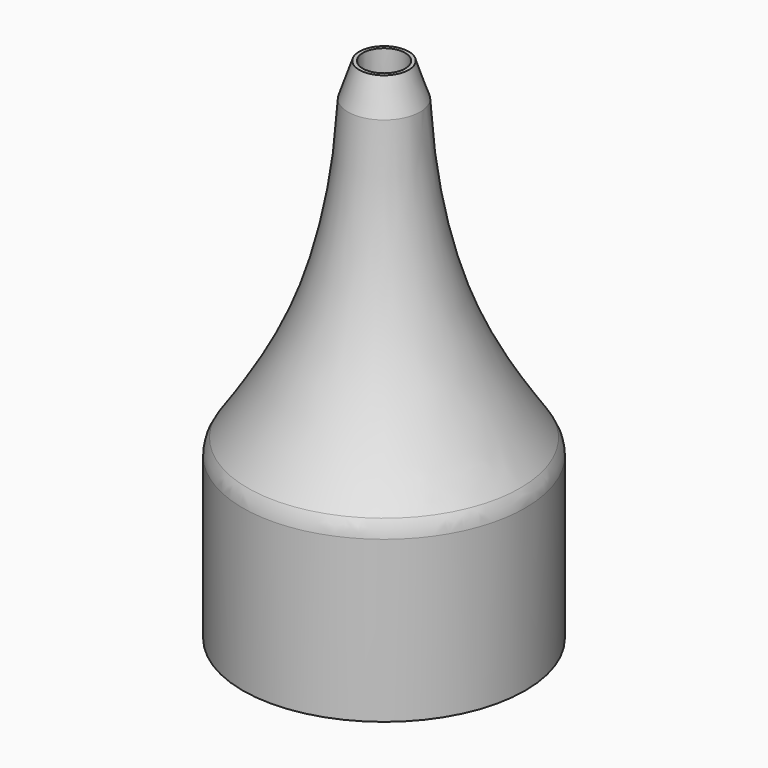
from build123d import *

# Parameters (mm, degrees)
F2_R = 6.35
F3_R = 3.175


# Not quite as in the source:
# - a fillet or chamfer that OpenCascade refuses, or shapes differently, is made with other operations: its cross-section is extruded or revolved along the edge and cut away or added


with BuildPart() as f1:
    # F0 (on Front) → F1 (revolve)
    with BuildSketch(Plane.XZ):
        with BuildLine():
            Line((28.575, 37.618366381), (28.575, 0))
            Line((28.575, 0), (31.75, 0))
            Line((31.75, 0), (31.75, 38.1))
            add(Edge.make_bspline(
                [(31.75, 38.1), (25.5696352748, 47.053791559), (12.6494179223, 66.7292187435), (7.9375, 97.4673148441), (7.9375, 114.3)],
                knots=[0, 0, 0, 0, 0.4558311814, 1, 1, 1, 1], degree=3))
            Line((7.9375, 114.3), (4.7625, 114.3))
            add(Edge.make_bspline(
                [(28.575, 37.618366381), (22.2120435784, 45.9360541366), (8.4198305726, 64.5807348307), (4.7625, 96.5429267445), (4.7625, 114.3)],
                knots=[0, 0, 0, 0, 0.4464692499, 1, 1, 1, 1], degree=3))
        make_face()
    revolve(axis=Axis((0, 0, 57.15), (0, 0, 1)))

    # F2
    f2_edges = [f1.edges().sort_by_distance(p)[0] for p in [
        (-31.75, 0, 38.1),
    ]]
    fillet(f2_edges, radius=F2_R)

    # F3
    f3_edges = [f1.edges().sort_by_distance(p)[0] for p in [
        (-28.575, 0, 37.618366),
    ]]
    fillet(f3_edges, radius=F3_R)

    # F4: chamfer of 7.62 x 2.54 on 1 edges, made by hand

    # F4_s1 → F4_t2 (revolve, cut)
    with BuildSketch(Plane.XZ):
        with BuildLine():
            Line((5.4727362401, 114.5887422704), (8.2053664291, 106.5066587943))
            Line((8.2053664291, 106.5066587943), (8.3576090556, 106.5135828582))
            ThreePointArc((8.3576090556, 106.5135828582), (8.1357267118, 110.4048430874), (8.0899, 114.3))
            Line((8.0899, 114.3), (7.9375, 114.4524))
            ThreePointArc((7.9375, 114.4524), (6.7051181201, 114.4524), (5.4727362401, 114.7411422704))
            Line((5.4727362401, 114.7411422704), (5.4727362401, 114.5887422704))
        make_face()
    revolve(axis=Axis((0, 0, 114.3), (0, 0, 1)), mode=Mode.SUBTRACT)


solid = f1.part
